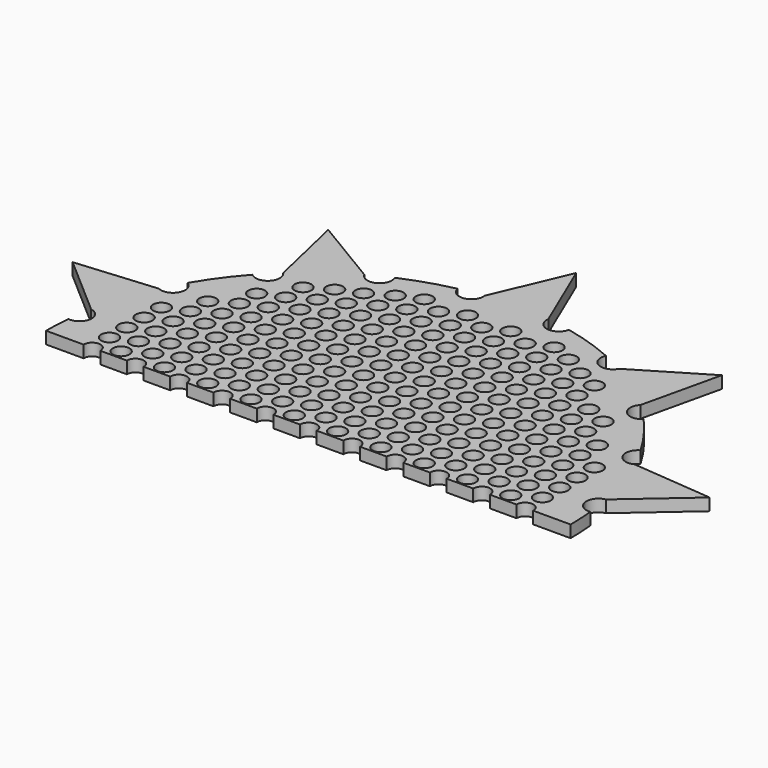
from build123d import *

# Parameters (mm, degrees)
F0_R     = 2.5
F1_DEPTH = 0.127
F3_R     = 0.0875
F4_DEPTH = 0.128
F5_W     = 8.2140588202
F5_H     = 3.6369306035
F6_DEPTH = 25


with BuildPart() as f1:
    # F0 (on Top) → F1 (new body)
    with BuildSketch(Plane.XY):
        with BuildLine():
            ThreePointArc((0.4371819273, 2.5863102989), (0.355691734, 2.6367647524), (0.332670369, 2.7298041002))
            ThreePointArc((0.332670369, 2.7298041002), (0, 2.75), (-0.332670369, 2.7298041002))
            ThreePointArc((-0.332670369, 2.7298041002), (-0.3556917334, 2.6367647532), (-0.4371819253, 2.5863102993))
            ThreePointArc((-0.4371819253, 2.5863102993), (1e-09, 2.623), (0.4371819273, 2.5863102989))
        make_face()
        with BuildLine():
            ThreePointArc((-0.332670369, 2.7298041002), (0, 2.75), (0.332670369, 2.7298041002))
            Line((0.332670369, 2.7298041002), (0, 3.512))
            Line((0, 3.512), (-0.332670369, 2.7298041002))
        make_face()
        with BuildLine():
            ThreePointArc((0.58305072, 2.6874805781), (0.5307280391, 2.6071771648), (0.4371819273, 2.5863102989))
            ThreePointArc((0.4371819273, 2.5863102989), (0.8105515843, 2.4946212396), (1.1665074579, 2.3493380665))
            ThreePointArc((1.1665074579, 2.3493380665), (1.1030922874, 2.4212047401), (1.1079635086, 2.5169260743))
            ThreePointArc((1.1079635086, 2.5169260743), (0.8497967345, 2.6154054198), (0.58305072, 2.6874805781))
        make_face()
        with BuildLine():
            ThreePointArc((1.1665074579, 2.3493380665), (0.8105515843, 2.4946212396), (0.4371819273, 2.5863102989))
            ThreePointArc((0.4371819273, 2.5863102989), (1e-09, 2.623), (-0.4371819253, 2.5863102993))
            ThreePointArc((-0.4371819253, 2.5863102993), (-0.8105515878, 2.4946212385), (-1.1665074663, 2.3493380623))
            ThreePointArc((-1.1665074663, 2.3493380623), (-1.5417607284, 2.1220515678), (-1.8738826621, 1.8353998934))
            ThreePointArc((-1.8738826621, 1.8353998934), (-2.1220515776, 1.5417607149), (-2.3246306188, 1.2149985539))
            ThreePointArc((-2.3246306188, 1.2149985539), (-2.4946212423, 0.8105515762), (-2.5948239078, 0.3834291163))
            ThreePointArc((-2.5948239078, 0.3834291163), (-2.623, 0), (-2.5948239078, -0.3834291163))
            ThreePointArc((-2.5948239078, -0.3834291163), (-2.4946212423, -0.8105515762), (-2.3246306188, -1.2149985539))
            ThreePointArc((-2.3246306188, -1.2149985539), (-2.1220515776, -1.5417607149), (-1.8738826621, -1.8353998934))
            ThreePointArc((-1.8738826621, -1.8353998934), (-1.5417607284, -2.1220515678), (-1.1665074663, -2.3493380623))
            ThreePointArc((-1.1665074663, -2.3493380623), (-0.8105515897, -2.4946212379), (-0.4371819293, -2.5863102986))
            ThreePointArc((-0.4371819293, -2.5863102986), (-1.56e-08, -2.623), (0.4371818986, -2.5863103038))
            ThreePointArc((0.4371818986, -2.5863103038), (0.8105515616, -2.494621247), (1.1665074412, -2.3493380748))
            ThreePointArc((1.1665074412, -2.3493380748), (1.541760707, -2.1220515834), (1.8738826446, -1.8353999112))
            ThreePointArc((1.8738826446, -1.8353999112), (2.1220515703, -1.541760725), (2.3246306188, -1.2149985539))
            ThreePointArc((2.3246306188, -1.2149985539), (2.4946212397, -0.8105515841), (2.5948239054, -0.3834291328))
            ThreePointArc((2.5948239054, -0.3834291328), (2.6159464926, -0.192231496), (2.623, 0))
            ThreePointArc((2.623, 0), (2.6159464926, 0.192231496), (2.5948239054, 0.3834291328))
            ThreePointArc((2.5948239054, 0.3834291328), (2.4946212397, 0.8105515841), (2.3246306188, 1.2149985539))
            ThreePointArc((2.3246306188, 1.2149985539), (2.1220515776, 1.5417607149), (1.8738826621, 1.8353998934))
            ThreePointArc((1.8738826621, 1.8353998934), (1.5417607246, 2.1220515706), (1.1665074579, 2.3493380665))
        make_face()
        Circle(F0_R, mode=Mode.SUBTRACT)
        with BuildLine():
            ThreePointArc((-1.1665074663, 2.3493380623), (-0.8105515878, 2.4946212385), (-0.4371819253, 2.5863102993))
            ThreePointArc((-0.4371819253, 2.5863102993), (-0.5307280383, 2.6071771643), (-0.58305072, 2.6874805781))
            ThreePointArc((-0.58305072, 2.6874805781), (-0.8497967345, 2.6154054198), (-1.1079635086, 2.5169260743))
            ThreePointArc((-1.1079635086, 2.5169260743), (-1.1030922889, 2.4212047357), (-1.1665074663, 2.3493380623))
        make_face()
        with BuildLine():
            ThreePointArc((1.3354026098, 2.4039966451), (1.2620907858, 2.3422578531), (1.1665074579, 2.3493380665))
            ThreePointArc((1.1665074579, 2.3493380665), (1.5417607246, 2.1220515706), (1.8738826621, 1.8353998934))
            ThreePointArc((1.8738826621, 1.8353998934), (1.8376120928, 1.9241171381), (1.8736745738, 2.0129191717))
            ThreePointArc((1.8736745738, 2.0129191717), (1.6164094438, 2.2247967345), (1.3354026098, 2.4039966451))
        make_face()
        with BuildLine():
            ThreePointArc((-1.8738826621, 1.8353998934), (-1.5417607284, 2.1220515678), (-1.1665074663, 2.3493380623))
            ThreePointArc((-1.1665074663, 2.3493380623), (-1.2620907902, 2.3422578545), (-1.3354026098, 2.4039966451))
            ThreePointArc((-1.3354026098, 2.4039966451), (-1.6164094438, 2.2247967345), (-1.8736745738, 2.0129191717))
            ThreePointArc((-1.8736745738, 2.0129191717), (-1.8376120928, 1.9241171381), (-1.8738826621, 1.8353998934))
        make_face()
        with BuildLine():
            ThreePointArc((2.0513593907, 1.8315088452), (1.9618282918, 1.7972965193), (1.8738826621, 1.8353998934))
            ThreePointArc((1.8738826621, 1.8353998934), (2.1220515776, 1.5417607149), (2.3246306188, 1.2149985539))
            ThreePointArc((2.3246306188, 1.2149985539), (2.315568848, 1.3104144102), (2.3757733352, 1.3849913573))
            ThreePointArc((2.3757733352, 1.3849913573), (2.2247967345, 1.6164094438), (2.0513593907, 1.8315088452))
        make_face()
        with BuildLine():
            Line((2.0643018061, 2.8412676842), (1.3354026098, 2.4039966451))
            ThreePointArc((1.3354026098, 2.4039966451), (1.6164094438, 2.2247967345), (1.8736745738, 2.0129191717))
            Line((1.8736745738, 2.0129191717), (2.0643018061, 2.8412676842))
        make_face()
        with BuildLine():
            ThreePointArc((-2.3246306188, 1.2149985539), (-2.1220515776, 1.5417607149), (-1.8738826621, 1.8353998934))
            ThreePointArc((-1.8738826621, 1.8353998934), (-1.9618282918, 1.7972965193), (-2.0513593907, 1.8315088452))
            ThreePointArc((-2.0513593907, 1.8315088452), (-2.2247967345, 1.6164094438), (-2.3757733352, 1.3849913573))
            ThreePointArc((-2.3757733352, 1.3849913573), (-2.315568848, 1.3104144102), (-2.3246306188, 1.2149985539))
        make_face()
        with BuildLine():
            ThreePointArc((-1.8736745738, 2.0129191717), (-1.6164094438, 2.2247967345), (-1.3354026098, 2.4039966451))
            Line((-1.3354026098, 2.4039966451), (-2.0643018061, 2.8412676842))
            Line((-2.0643018061, 2.8412676842), (-1.8736745738, 2.0129191717))
        make_face()
        with BuildLine():
            ThreePointArc((2.4933971802, 1.1599441805), (2.3977975102, 1.1530880597), (2.3246306188, 1.2149985539))
            ThreePointArc((2.3246306188, 1.2149985539), (2.4946212397, 0.8105515841), (2.5948239054, 0.3834291328))
            ThreePointArc((2.5948239054, 0.3834291328), (2.6176270957, 0.4765221848), (2.6989987753, 0.5271675361))
            ThreePointArc((2.6989987753, 0.5271675361), (2.6154054198, 0.8497967345), (2.4933971802, 1.1599441805))
        make_face()
        with BuildLine():
            ThreePointArc((-2.5948239078, 0.3834291163), (-2.4946212423, 0.8105515762), (-2.3246306188, 1.2149985539))
            ThreePointArc((-2.3246306188, 1.2149985539), (-2.3977975102, 1.1530880597), (-2.4933971802, 1.1599441805))
            ThreePointArc((-2.4933971802, 1.1599441805), (-2.6154054198, 0.8497967345), (-2.6989987753, 0.5271675361))
            ThreePointArc((-2.6989987753, 0.5271675361), (-2.6176270909, 0.4765221781), (-2.5948239078, 0.3834291163))
        make_face()
        with BuildLine():
            ThreePointArc((2.7361184973, 0.2759629841), (2.6435768078, 0.300909697), (2.5948239054, 0.3834291328))
            ThreePointArc((2.5948239054, 0.3834291328), (2.6159464926, 0.192231496), (2.623, 0))
            ThreePointArc((2.623, 0), (2.6159464926, -0.192231496), (2.5948239054, -0.3834291328))
            ThreePointArc((2.5948239054, -0.3834291328), (2.6435768078, -0.300909697), (2.7361184973, -0.2759629841))
            ThreePointArc((2.7361184973, -0.2759629841), (2.75, 0), (2.7361184973, 0.2759629841))
        make_face()
        with BuildLine():
            Line((3.3401104852, 1.0852676842), (2.4933971802, 1.1599441805))
            ThreePointArc((2.4933971802, 1.1599441805), (2.6154054198, 0.8497967345), (2.6989987753, 0.5271675361))
            Line((2.6989987753, 0.5271675361), (3.3401104852, 1.0852676842))
        make_face()
        with BuildLine():
            ThreePointArc((-2.5948239078, -0.3834291163), (-2.623, 0), (-2.5948239078, 0.3834291163))
            ThreePointArc((-2.5948239078, 0.3834291163), (-2.6435768144, 0.3009096919), (-2.7361184973, 0.2759629841))
            ThreePointArc((-2.7361184973, 0.2759629841), (-2.75, 0), (-2.7361184973, -0.2759629841))
            ThreePointArc((-2.7361184973, -0.2759629841), (-2.6435768144, -0.3009096919), (-2.5948239078, -0.3834291163))
        make_face()
        with BuildLine():
            ThreePointArc((-2.6989987753, 0.5271675361), (-2.6154054198, 0.8497967345), (-2.4933971802, 1.1599441805))
            Line((-2.4933971802, 1.1599441805), (-3.3401104852, 1.0852676842))
            Line((-3.3401104852, 1.0852676842), (-2.6989987753, 0.5271675361))
        make_face()
        with BuildLine():
            ThreePointArc((-2.3246306188, -1.2149985539), (-2.4946212423, -0.8105515762), (-2.5948239078, -0.3834291163))
            ThreePointArc((-2.5948239078, -0.3834291163), (-2.6176270909, -0.4765221781), (-2.6989987753, -0.5271675361))
            ThreePointArc((-2.6989987753, -0.5271675361), (-2.6154054198, -0.8497967345), (-2.4933971802, -1.1599441805))
            ThreePointArc((-2.4933971802, -1.1599441805), (-2.3977975102, -1.1530880597), (-2.3246306188, -1.2149985539))
        make_face()
        with BuildLine():
            ThreePointArc((2.6989987753, -0.5271675361), (2.6176270957, -0.4765221848), (2.5948239054, -0.3834291328))
            ThreePointArc((2.5948239054, -0.3834291328), (2.4946212397, -0.8105515841), (2.3246306188, -1.2149985539))
            ThreePointArc((2.3246306188, -1.2149985539), (2.3977975102, -1.1530880597), (2.4933971802, -1.1599441805))
            ThreePointArc((2.4933971802, -1.1599441805), (2.6154054198, -0.8497967345), (2.6989987753, -0.5271675361))
        make_face()
        with BuildLine():
            ThreePointArc((-1.8738826621, -1.8353998934), (-2.1220515776, -1.5417607149), (-2.3246306188, -1.2149985539))
            ThreePointArc((-2.3246306188, -1.2149985539), (-2.315568848, -1.3104144102), (-2.3757733352, -1.3849913573))
            ThreePointArc((-2.3757733352, -1.3849913573), (-2.2247967345, -1.6164094438), (-2.0513593907, -1.8315088452))
            ThreePointArc((-2.0513593907, -1.8315088452), (-1.9618282918, -1.7972965193), (-1.8738826621, -1.8353998934))
        make_face()
        with BuildLine():
            ThreePointArc((-2.4933971802, -1.1599441805), (-2.6154054198, -0.8497967345), (-2.6989987753, -0.5271675361))
            Line((-2.6989987753, -0.5271675361), (-3.3401104852, -1.0852676842))
            Line((-3.3401104852, -1.0852676842), (-2.4933971802, -1.1599441805))
        make_face()
        with BuildLine():
            ThreePointArc((2.3757733352, -1.3849913573), (2.315568848, -1.3104144102), (2.3246306188, -1.2149985539))
            ThreePointArc((2.3246306188, -1.2149985539), (2.1220515703, -1.541760725), (1.8738826446, -1.8353999112))
            ThreePointArc((1.8738826446, -1.8353999112), (1.9618282794, -1.7972965196), (2.0513593907, -1.8315088452))
            ThreePointArc((2.0513593907, -1.8315088452), (2.2247967345, -1.6164094438), (2.3757733352, -1.3849913573))
        make_face()
        with BuildLine():
            Line((3.3401104852, -1.0852676842), (2.6989987753, -0.5271675361))
            ThreePointArc((2.6989987753, -0.5271675361), (2.6154054198, -0.8497967345), (2.4933971802, -1.1599441805))
            Line((2.4933971802, -1.1599441805), (3.3401104852, -1.0852676842))
        make_face()
        with BuildLine():
            ThreePointArc((-1.1665074663, -2.3493380623), (-1.5417607284, -2.1220515678), (-1.8738826621, -1.8353998934))
            ThreePointArc((-1.8738826621, -1.8353998934), (-1.8376120928, -1.9241171381), (-1.8736745738, -2.0129191717))
            ThreePointArc((-1.8736745738, -2.0129191717), (-1.6164094438, -2.2247967345), (-1.3354026098, -2.4039966451))
            ThreePointArc((-1.3354026098, -2.4039966451), (-1.2620907902, -2.3422578545), (-1.1665074663, -2.3493380623))
        make_face()
        with BuildLine():
            ThreePointArc((1.8736745738, -2.0129191717), (1.8376120928, -1.9241171506), (1.8738826446, -1.8353999112))
            ThreePointArc((1.8738826446, -1.8353999112), (1.541760707, -2.1220515834), (1.1665074412, -2.3493380748))
            ThreePointArc((1.1665074412, -2.3493380748), (1.2620907769, -2.3422578502), (1.3354026098, -2.4039966451))
            ThreePointArc((1.3354026098, -2.4039966451), (1.6164094438, -2.2247967345), (1.8736745738, -2.0129191717))
        make_face()
        with BuildLine():
            ThreePointArc((-0.4371819293, -2.5863102986), (-0.8105515897, -2.4946212379), (-1.1665074663, -2.3493380623))
            ThreePointArc((-1.1665074663, -2.3493380623), (-1.1030922889, -2.4212047357), (-1.1079635086, -2.5169260743))
            ThreePointArc((-1.1079635086, -2.5169260743), (-0.8497967345, -2.6154054198), (-0.58305072, -2.6874805781))
            ThreePointArc((-0.58305072, -2.6874805781), (-0.5307280399, -2.6071771654), (-0.4371819293, -2.5863102986))
        make_face()
        with BuildLine():
            ThreePointArc((-1.3354026098, -2.4039966451), (-1.6164094438, -2.2247967345), (-1.8736745738, -2.0129191717))
            Line((-1.8736745738, -2.0129191717), (-2.0643018061, -2.8412676842))
            Line((-2.0643018061, -2.8412676842), (-1.3354026098, -2.4039966451))
        make_face()
        with BuildLine():
            ThreePointArc((1.1079635086, -2.5169260743), (1.1030922843, -2.4212047489), (1.1665074412, -2.3493380748))
            ThreePointArc((1.1665074412, -2.3493380748), (0.8105515616, -2.494621247), (0.4371818986, -2.5863103038))
            ThreePointArc((0.4371818986, -2.5863103038), (0.5307280271, -2.6071771565), (0.58305072, -2.6874805781))
            ThreePointArc((0.58305072, -2.6874805781), (0.8497967345, -2.6154054198), (1.1079635086, -2.5169260743))
        make_face()
        with BuildLine():
            Line((2.0643018061, -2.8412676842), (1.8736745738, -2.0129191717))
            ThreePointArc((1.8736745738, -2.0129191717), (1.6164094438, -2.2247967345), (1.3354026098, -2.4039966451))
            Line((1.3354026098, -2.4039966451), (2.0643018061, -2.8412676842))
        make_face()
        with BuildLine():
            ThreePointArc((0.4371818986, -2.5863103038), (-1.56e-08, -2.623), (-0.4371819293, -2.5863102986))
            ThreePointArc((-0.4371819293, -2.5863102986), (-0.3556917345, -2.6367647516), (-0.332670369, -2.7298041002))
            ThreePointArc((-0.332670369, -2.7298041002), (0, -2.75), (0.332670369, -2.7298041002))
            ThreePointArc((0.332670369, -2.7298041002), (0.3556917254, -2.6367647642), (0.4371818986, -2.5863103038))
        make_face()
        with BuildLine():
            ThreePointArc((0.332670369, -2.7298041002), (0, -2.75), (-0.332670369, -2.7298041002))
            Line((-0.332670369, -2.7298041002), (0, -3.512))
            Line((0, -3.512), (0.332670369, -2.7298041002))
        make_face()
        Circle(F0_R)
    extrude(amount=F1_DEPTH)

    # F3 (on offset) → F4 (cut, through all)
    with BuildSketch(Plane.XY.offset(0.127)):
        with Locations((-2.0417519944, 1.2336155081)):
            Circle(F3_R)
        with Locations((-2.0417519944, 1.0066155081)):
            Circle(F3_R)
        with Locations((-2.2690836629, 0.9108655081)):
            Circle(F3_R)
        with Locations((-2.0417519944, 0.7796155081)):
            Circle(F3_R)
        with Locations((-1.5877519944, 1.9146155081)):
            Circle(F3_R)
        with Locations((-1.5877519944, 1.6876155081)):
            Circle(F3_R)
        with Locations((-1.8150836629, 1.5918655081)):
            Circle(F3_R)
        with Locations((-1.5877519944, 1.4606155081)):
            Circle(F3_R)
        with Locations((-1.8150836629, 1.3648655081)):
            Circle(F3_R)
        with Locations((-1.5877519944, 1.2336155081)):
            Circle(F3_R)
        with Locations((-1.8150836629, 1.1378655081)):
            Circle(F3_R)
        with Locations((-1.5877519944, 1.0066155081)):
            Circle(F3_R)
        with Locations((-1.8150836629, 0.9108655081)):
            Circle(F3_R)
        with Locations((-1.5877519944, 0.7796155081)):
            Circle(F3_R)
        with Locations((-1.1337519944, 2.1416155081)):
            Circle(F3_R)
        with Locations((-1.3610836629, 2.0458655081)):
            Circle(F3_R)
        with Locations((-1.1337519944, 1.9146155081)):
            Circle(F3_R)
        with Locations((-1.3610836629, 1.8188655081)):
            Circle(F3_R)
        with Locations((-1.1337519944, 1.6876155081)):
            Circle(F3_R)
        with Locations((-1.3610836629, 1.5918655081)):
            Circle(F3_R)
        with Locations((-1.1337519944, 1.4606155081)):
            Circle(F3_R)
        with Locations((-1.3610836629, 1.3648655081)):
            Circle(F3_R)
        with Locations((-1.1337519944, 1.2336155081)):
            Circle(F3_R)
        with Locations((-1.3610836629, 1.1378655081)):
            Circle(F3_R)
        with Locations((-1.1337519944, 1.0066155081)):
            Circle(F3_R)
        with Locations((-1.3610836629, 0.9108655081)):
            Circle(F3_R)
        with Locations((-1.1337519944, 0.7796155081)):
            Circle(F3_R)
        with Locations((-0.6797519944, 2.3686155081)):
            Circle(F3_R)
        with Locations((-0.9070836629, 2.2728655081)):
            Circle(F3_R)
        with Locations((-0.6797519944, 2.1416155081)):
            Circle(F3_R)
        with Locations((-0.9070836629, 2.0458655081)):
            Circle(F3_R)
        with Locations((-0.6797519944, 1.9146155081)):
            Circle(F3_R)
        with Locations((-0.9070836629, 1.8188655081)):
            Circle(F3_R)
        with Locations((-0.6797519944, 1.6876155081)):
            Circle(F3_R)
        with Locations((-0.9070836629, 1.5918655081)):
            Circle(F3_R)
        with Locations((-0.6797519944, 1.4606155081)):
            Circle(F3_R)
        with Locations((-0.9070836629, 1.3648655081)):
            Circle(F3_R)
        with Locations((-0.6797519944, 1.2336155081)):
            Circle(F3_R)
        with Locations((-0.9070836629, 1.1378655081)):
            Circle(F3_R)
        with Locations((-0.6797519944, 1.0066155081)):
            Circle(F3_R)
        with Locations((-0.9070836629, 0.9108655081)):
            Circle(F3_R)
        with Locations((-0.6797519944, 0.7796155081)):
            Circle(F3_R)
        with Locations((-0.2257519944, 2.3686155081)):
            Circle(F3_R)
        with Locations((-0.4530836629, 2.2728655081)):
            Circle(F3_R)
        with Locations((-0.2257519944, 2.1416155081)):
            Circle(F3_R)
        with Locations((-0.4530836629, 2.0458655081)):
            Circle(F3_R)
        with Locations((-0.2257519944, 1.9146155081)):
            Circle(F3_R)
        with Locations((-0.4530836629, 1.8188655081)):
            Circle(F3_R)
        with Locations((-0.2257519944, 1.6876155081)):
            Circle(F3_R)
        with Locations((-0.4530836629, 1.5918655081)):
            Circle(F3_R)
        with Locations((-0.2257519944, 1.4606155081)):
            Circle(F3_R)
        with Locations((-0.4530836629, 1.3648655081)):
            Circle(F3_R)
        with Locations((-0.2257519944, 1.2336155081)):
            Circle(F3_R)
        with Locations((-0.4530836629, 1.1378655081)):
            Circle(F3_R)
        with Locations((-0.2257519944, 1.0066155081)):
            Circle(F3_R)
        with Locations((-0.4530836629, 0.9108655081)):
            Circle(F3_R)
        with Locations((-0.2257519944, 0.7796155081)):
            Circle(F3_R)
        with Locations((0.2282480056, 2.3686155081)):
            Circle(F3_R)
        with Locations((0.0009163371, 2.2728655081)):
            Circle(F3_R)
        with Locations((0.2282480056, 2.1416155081)):
            Circle(F3_R)
        with Locations((0.0009163371, 2.0458655081)):
            Circle(F3_R)
        with Locations((0.2282480056, 1.9146155081)):
            Circle(F3_R)
        with Locations((0.0009163371, 1.8188655081)):
            Circle(F3_R)
        with Locations((0.2282480056, 1.6876155081)):
            Circle(F3_R)
        with Locations((0.0009163371, 1.5918655081)):
            Circle(F3_R)
        with Locations((0.2282480056, 1.4606155081)):
            Circle(F3_R)
        with Locations((0.0009163371, 1.3648655081)):
            Circle(F3_R)
        with Locations((0.2282480056, 1.2336155081)):
            Circle(F3_R)
        with Locations((0.0009163371, 1.1378655081)):
            Circle(F3_R)
        with Locations((0.2282480056, 1.0066155081)):
            Circle(F3_R)
        with Locations((0.0009163371, 0.9108655081)):
            Circle(F3_R)
        with Locations((0.2282480056, 0.7796155081)):
            Circle(F3_R)
        with Locations((0.6822480056, 2.3686155081)):
            Circle(F3_R)
        with Locations((0.4549163371, 2.2728655081)):
            Circle(F3_R)
        with Locations((0.6822480056, 2.1416155081)):
            Circle(F3_R)
        with Locations((0.4549163371, 2.0458655081)):
            Circle(F3_R)
        with Locations((0.6822480056, 1.9146155081)):
            Circle(F3_R)
        with Locations((0.4549163371, 1.8188655081)):
            Circle(F3_R)
        with Locations((0.6822480056, 1.6876155081)):
            Circle(F3_R)
        with Locations((0.4549163371, 1.5918655081)):
            Circle(F3_R)
        with Locations((0.6822480056, 1.4606155081)):
            Circle(F3_R)
        with Locations((0.4549163371, 1.3648655081)):
            Circle(F3_R)
        with Locations((0.6822480056, 1.2336155081)):
            Circle(F3_R)
        with Locations((0.4549163371, 1.1378655081)):
            Circle(F3_R)
        with Locations((0.6822480056, 1.0066155081)):
            Circle(F3_R)
        with Locations((0.4549163371, 0.9108655081)):
            Circle(F3_R)
        with Locations((0.6822480056, 0.7796155081)):
            Circle(F3_R)
        with Locations((0.9089163371, 2.2728655081)):
            Circle(F3_R)
        with Locations((1.1362480056, 2.1416155081)):
            Circle(F3_R)
        with Locations((0.9089163371, 2.0458655081)):
            Circle(F3_R)
        with Locations((1.1362480056, 1.9146155081)):
            Circle(F3_R)
        with Locations((0.9089163371, 1.8188655081)):
            Circle(F3_R)
        with Locations((1.1362480056, 1.6876155081)):
            Circle(F3_R)
        with Locations((0.9089163371, 1.5918655081)):
            Circle(F3_R)
        with Locations((1.1362480056, 1.4606155081)):
            Circle(F3_R)
        with Locations((0.9089163371, 1.3648655081)):
            Circle(F3_R)
        with Locations((1.1362480056, 1.2336155081)):
            Circle(F3_R)
        with Locations((0.9089163371, 1.1378655081)):
            Circle(F3_R)
        with Locations((1.1362480056, 1.0066155081)):
            Circle(F3_R)
        with Locations((0.9089163371, 0.9108655081)):
            Circle(F3_R)
        with Locations((1.1362480056, 0.7796155081)):
            Circle(F3_R)
        with Locations((1.3629163371, 2.0458655081)):
            Circle(F3_R)
        with Locations((1.3629163371, 1.8188655081)):
            Circle(F3_R)
        with Locations((1.5902480056, 1.6876155081)):
            Circle(F3_R)
        with Locations((1.3629163371, 1.5918655081)):
            Circle(F3_R)
        with Locations((1.5902480056, 1.4606155081)):
            Circle(F3_R)
        with Locations((1.3629163371, 1.3648655081)):
            Circle(F3_R)
        with Locations((1.5902480056, 1.2336155081)):
            Circle(F3_R)
        with Locations((1.3629163371, 1.1378655081)):
            Circle(F3_R)
        with Locations((1.5902480056, 1.0066155081)):
            Circle(F3_R)
        with Locations((1.3629163371, 0.9108655081)):
            Circle(F3_R)
        with Locations((1.5902480056, 0.7796155081)):
            Circle(F3_R)
        with Locations((1.8169163371, 1.5918655081)):
            Circle(F3_R)
        with Locations((1.8169163371, 1.3648655081)):
            Circle(F3_R)
        with Locations((2.0442480056, 1.2336155081)):
            Circle(F3_R)
        with Locations((1.8169163371, 1.1378655081)):
            Circle(F3_R)
        with Locations((2.0442480056, 1.0066155081)):
            Circle(F3_R)
        with Locations((1.8169163371, 0.9108655081)):
            Circle(F3_R)
        with Locations((2.0442480056, 0.7796155081)):
            Circle(F3_R)
        with Locations((-2.2690836629, 0.6838655081)):
            Circle(F3_R)
        with Locations((-2.0417519944, 0.5526155081)):
            Circle(F3_R)
        with Locations((-2.2690836629, 0.4568655081)):
            Circle(F3_R)
        with Locations((-2.0417519944, 0.3256155081)):
            Circle(F3_R)
        with Locations((-2.2690836629, 0.2298655081)):
            Circle(F3_R)
        with Locations((-2.0417519944, 0.0986155081)):
            Circle(F3_R)
        with Locations((-2.2690836629, 0.0028655081)):
            Circle(F3_R)
        with Locations((-2.0417519944, -0.1283844919)):
            Circle(F3_R)
        with Locations((-2.2690836629, -0.2241344919)):
            Circle(F3_R)
        with Locations((-2.0417519944, -0.3553844919)):
            Circle(F3_R)
        with Locations((-2.2690836629, -0.4511344919)):
            Circle(F3_R)
        with Locations((-2.0417519944, -0.5823844919)):
            Circle(F3_R)
        with Locations((-2.2690836629, -0.6781344919)):
            Circle(F3_R)
        with Locations((-2.0417519944, -0.8093844919)):
            Circle(F3_R)
        with Locations((-2.2690836629, -0.9051344919)):
            Circle(F3_R)
        with Locations((-2.0417519944, -1.0363844919)):
            Circle(F3_R)
        with Locations((-2.0417519944, -1.2633844919)):
            Circle(F3_R)
        with Locations((-1.8150836629, 0.6838655081)):
            Circle(F3_R)
        with Locations((-1.5877519944, 0.5526155081)):
            Circle(F3_R)
        with Locations((-1.8150836629, 0.4568655081)):
            Circle(F3_R)
        with Locations((-1.5877519944, 0.3256155081)):
            Circle(F3_R)
        with Locations((-1.8150836629, 0.2298655081)):
            Circle(F3_R)
        with Locations((-1.5877519944, 0.0986155081)):
            Circle(F3_R)
        with Locations((-1.8150836629, 0.0028655081)):
            Circle(F3_R)
        with Locations((-1.5877519944, -0.1283844919)):
            Circle(F3_R)
        with Locations((-1.8150836629, -0.2241344919)):
            Circle(F3_R)
        with Locations((-1.5877519944, -0.3553844919)):
            Circle(F3_R)
        with Locations((-1.8150836629, -0.4511344919)):
            Circle(F3_R)
        with Locations((-1.5877519944, -0.5823844919)):
            Circle(F3_R)
        with Locations((-1.8150836629, -0.6781344919)):
            Circle(F3_R)
        with Locations((-1.5877519944, -0.8093844919)):
            Circle(F3_R)
        with Locations((-1.8150836629, -0.9051344919)):
            Circle(F3_R)
        with Locations((-1.5877519944, -1.0363844919)):
            Circle(F3_R)
        with Locations((-1.8150836629, -1.1321344919)):
            Circle(F3_R)
        with Locations((-1.5877519944, -1.2633844919)):
            Circle(F3_R)
        with Locations((-1.8150836629, -1.3591344919)):
            Circle(F3_R)
        with Locations((-1.5877519944, -1.4903844919)):
            Circle(F3_R)
        with Locations((-1.8150836629, -1.5861344919)):
            Circle(F3_R)
        with Locations((-1.5877519944, -1.7173844919)):
            Circle(F3_R)
        with Locations((-1.3610836629, 0.6838655081)):
            Circle(F3_R)
        with Locations((-1.1337519944, 0.5526155081)):
            Circle(F3_R)
        with Locations((-1.3610836629, 0.4568655081)):
            Circle(F3_R)
        with Locations((-1.1337519944, 0.3256155081)):
            Circle(F3_R)
        with Locations((-1.3610836629, 0.2298655081)):
            Circle(F3_R)
        with Locations((-1.1337519944, 0.0986155081)):
            Circle(F3_R)
        with Locations((-1.3610836629, 0.0028655081)):
            Circle(F3_R)
        with Locations((-1.1337519944, -0.1283844919)):
            Circle(F3_R)
        with Locations((-1.3610836629, -0.2241344919)):
            Circle(F3_R)
        with Locations((-1.1337519944, -0.3553844919)):
            Circle(F3_R)
        with Locations((-1.3610836629, -0.4511344919)):
            Circle(F3_R)
        with Locations((-1.1337519944, -0.5823844919)):
            Circle(F3_R)
        with Locations((-1.3610836629, -0.6781344919)):
            Circle(F3_R)
        with Locations((-1.1337519944, -0.8093844919)):
            Circle(F3_R)
        with Locations((-1.3610836629, -0.9051344919)):
            Circle(F3_R)
        with Locations((-1.1337519944, -1.0363844919)):
            Circle(F3_R)
        with Locations((-1.3610836629, -1.1321344919)):
            Circle(F3_R)
        with Locations((-1.1337519944, -1.2633844919)):
            Circle(F3_R)
        with Locations((-1.3610836629, -1.3591344919)):
            Circle(F3_R)
        with Locations((-1.1337519944, -1.4903844919)):
            Circle(F3_R)
        with Locations((-1.3610836629, -1.5861344919)):
            Circle(F3_R)
        with Locations((-1.1337519944, -1.7173844919)):
            Circle(F3_R)
        with Locations((-0.9070836629, 0.6838655081)):
            Circle(F3_R)
        with Locations((-0.6797519944, 0.5526155081)):
            Circle(F3_R)
        with Locations((-0.9070836629, 0.4568655081)):
            Circle(F3_R)
        with Locations((-0.6797519944, 0.3256155081)):
            Circle(F3_R)
        with Locations((-0.9070836629, 0.2298655081)):
            Circle(F3_R)
        with Locations((-0.6797519944, 0.0986155081)):
            Circle(F3_R)
        with Locations((-0.9070836629, 0.0028655081)):
            Circle(F3_R)
        with Locations((-0.6797519944, -0.1283844919)):
            Circle(F3_R)
        with Locations((-0.9070836629, -0.2241344919)):
            Circle(F3_R)
        with Locations((-0.6797519944, -0.3553844919)):
            Circle(F3_R)
        with Locations((-0.9070836629, -0.4511344919)):
            Circle(F3_R)
        with Locations((-0.6797519944, -0.5823844919)):
            Circle(F3_R)
        with Locations((-0.9070836629, -0.6781344919)):
            Circle(F3_R)
        with Locations((-0.6797519944, -0.8093844919)):
            Circle(F3_R)
        with Locations((-0.9070836629, -0.9051344919)):
            Circle(F3_R)
        with Locations((-0.6797519944, -1.0363844919)):
            Circle(F3_R)
        with Locations((-0.9070836629, -1.1321344919)):
            Circle(F3_R)
        with Locations((-0.6797519944, -1.2633844919)):
            Circle(F3_R)
        with Locations((-0.9070836629, -1.3591344919)):
            Circle(F3_R)
        with Locations((-0.6797519944, -1.4903844919)):
            Circle(F3_R)
        with Locations((-0.9070836629, -1.5861344919)):
            Circle(F3_R)
        with Locations((-0.6797519944, -1.7173844919)):
            Circle(F3_R)
        with Locations((-0.4530836629, 0.6838655081)):
            Circle(F3_R)
        with Locations((-0.2257519944, 0.5526155081)):
            Circle(F3_R)
        with Locations((-0.4530836629, 0.4568655081)):
            Circle(F3_R)
        with Locations((-0.2257519944, 0.3256155081)):
            Circle(F3_R)
        with Locations((-0.4530836629, 0.2298655081)):
            Circle(F3_R)
        with Locations((-0.2257519944, 0.0986155081)):
            Circle(F3_R)
        with Locations((-0.4530836629, 0.0028655081)):
            Circle(F3_R)
        with Locations((-0.2257519944, -0.1283844919)):
            Circle(F3_R)
        with Locations((-0.4530836629, -0.2241344919)):
            Circle(F3_R)
        with Locations((-0.2257519944, -0.3553844919)):
            Circle(F3_R)
        with Locations((-0.4530836629, -0.4511344919)):
            Circle(F3_R)
        with Locations((-0.2257519944, -0.5823844919)):
            Circle(F3_R)
        with Locations((-0.4530836629, -0.6781344919)):
            Circle(F3_R)
        with Locations((-0.2257519944, -0.8093844919)):
            Circle(F3_R)
        with Locations((-0.4530836629, -0.9051344919)):
            Circle(F3_R)
        with Locations((-0.2257519944, -1.0363844919)):
            Circle(F3_R)
        with Locations((-0.4530836629, -1.1321344919)):
            Circle(F3_R)
        with Locations((-0.2257519944, -1.2633844919)):
            Circle(F3_R)
        with Locations((-0.4530836629, -1.3591344919)):
            Circle(F3_R)
        with Locations((-0.2257519944, -1.4903844919)):
            Circle(F3_R)
        with Locations((-0.4530836629, -1.5861344919)):
            Circle(F3_R)
        with Locations((-0.2257519944, -1.7173844919)):
            Circle(F3_R)
        with Locations((0.0009163371, 0.6838655081)):
            Circle(F3_R)
        with Locations((0.2282480056, 0.5526155081)):
            Circle(F3_R)
        with Locations((0.0009163371, 0.4568655081)):
            Circle(F3_R)
        with Locations((0.2282480056, 0.3256155081)):
            Circle(F3_R)
        with Locations((0.0009163371, 0.2298655081)):
            Circle(F3_R)
        with Locations((0.2282480056, 0.0986155081)):
            Circle(F3_R)
        with Locations((0.0009163371, 0.0028655081)):
            Circle(F3_R)
        with Locations((0.2282480056, -0.1283844919)):
            Circle(F3_R)
        with Locations((0.0009163371, -0.2241344919)):
            Circle(F3_R)
        with Locations((0.2282480056, -0.3553844919)):
            Circle(F3_R)
        with Locations((0.0009163371, -0.4511344919)):
            Circle(F3_R)
        with Locations((0.2282480056, -0.5823844919)):
            Circle(F3_R)
        with Locations((0.0009163371, -0.6781344919)):
            Circle(F3_R)
        with Locations((0.2282480056, -0.8093844919)):
            Circle(F3_R)
        with Locations((0.0009163371, -0.9051344919)):
            Circle(F3_R)
        with Locations((0.2282480056, -1.0363844919)):
            Circle(F3_R)
        with Locations((0.0009163371, -1.1321344919)):
            Circle(F3_R)
        with Locations((0.2282480056, -1.2633844919)):
            Circle(F3_R)
        with Locations((0.0009163371, -1.3591344919)):
            Circle(F3_R)
        with Locations((0.2282480056, -1.4903844919)):
            Circle(F3_R)
        with Locations((0.0009163371, -1.5861344919)):
            Circle(F3_R)
        with Locations((0.2282480056, -1.7173844919)):
            Circle(F3_R)
        with Locations((0.4549163371, 0.6838655081)):
            Circle(F3_R)
        with Locations((0.6822480056, 0.5526155081)):
            Circle(F3_R)
        with Locations((0.4549163371, 0.4568655081)):
            Circle(F3_R)
        with Locations((0.6822480056, 0.3256155081)):
            Circle(F3_R)
        with Locations((0.4549163371, 0.2298655081)):
            Circle(F3_R)
        with Locations((0.6822480056, 0.0986155081)):
            Circle(F3_R)
        with Locations((0.4549163371, 0.0028655081)):
            Circle(F3_R)
        with Locations((0.6822480056, -0.1283844919)):
            Circle(F3_R)
        with Locations((0.4549163371, -0.2241344919)):
            Circle(F3_R)
        with Locations((0.6822480056, -0.3553844919)):
            Circle(F3_R)
        with Locations((0.4549163371, -0.4511344919)):
            Circle(F3_R)
        with Locations((0.6822480056, -0.5823844919)):
            Circle(F3_R)
        with Locations((0.4549163371, -0.6781344919)):
            Circle(F3_R)
        with Locations((0.6822480056, -0.8093844919)):
            Circle(F3_R)
        with Locations((0.4549163371, -0.9051344919)):
            Circle(F3_R)
        with Locations((0.6822480056, -1.0363844919)):
            Circle(F3_R)
        with Locations((0.4549163371, -1.1321344919)):
            Circle(F3_R)
        with Locations((0.6822480056, -1.2633844919)):
            Circle(F3_R)
        with Locations((0.4549163371, -1.3591344919)):
            Circle(F3_R)
        with Locations((0.6822480056, -1.4903844919)):
            Circle(F3_R)
        with Locations((0.4549163371, -1.5861344919)):
            Circle(F3_R)
        with Locations((0.6822480056, -1.7173844919)):
            Circle(F3_R)
        with Locations((0.9089163371, 0.6838655081)):
            Circle(F3_R)
        with Locations((1.1362480056, 0.5526155081)):
            Circle(F3_R)
        with Locations((0.9089163371, 0.4568655081)):
            Circle(F3_R)
        with Locations((1.1362480056, 0.3256155081)):
            Circle(F3_R)
        with Locations((0.9089163371, 0.2298655081)):
            Circle(F3_R)
        with Locations((1.1362480056, 0.0986155081)):
            Circle(F3_R)
        with Locations((0.9089163371, 0.0028655081)):
            Circle(F3_R)
        with Locations((1.1362480056, -0.1283844919)):
            Circle(F3_R)
        with Locations((0.9089163371, -0.2241344919)):
            Circle(F3_R)
        with Locations((1.1362480056, -0.3553844919)):
            Circle(F3_R)
        with Locations((0.9089163371, -0.4511344919)):
            Circle(F3_R)
        with Locations((1.1362480056, -0.5823844919)):
            Circle(F3_R)
        with Locations((0.9089163371, -0.6781344919)):
            Circle(F3_R)
        with Locations((1.1362480056, -0.8093844919)):
            Circle(F3_R)
        with Locations((0.9089163371, -0.9051344919)):
            Circle(F3_R)
        with Locations((1.1362480056, -1.0363844919)):
            Circle(F3_R)
        with Locations((0.9089163371, -1.1321344919)):
            Circle(F3_R)
        with Locations((1.1362480056, -1.2633844919)):
            Circle(F3_R)
        with Locations((0.9089163371, -1.3591344919)):
            Circle(F3_R)
        with Locations((1.1362480056, -1.4903844919)):
            Circle(F3_R)
        with Locations((0.9089163371, -1.5861344919)):
            Circle(F3_R)
        with Locations((1.1362480056, -1.7173844919)):
            Circle(F3_R)
        with Locations((1.3629163371, 0.6838655081)):
            Circle(F3_R)
        with Locations((1.5902480056, 0.5526155081)):
            Circle(F3_R)
        with Locations((1.3629163371, 0.4568655081)):
            Circle(F3_R)
        with Locations((1.5902480056, 0.3256155081)):
            Circle(F3_R)
        with Locations((1.3629163371, 0.2298655081)):
            Circle(F3_R)
        with Locations((1.5902480056, 0.0986155081)):
            Circle(F3_R)
        with Locations((1.3629163371, 0.0028655081)):
            Circle(F3_R)
        with Locations((1.5902480056, -0.1283844919)):
            Circle(F3_R)
        with Locations((1.3629163371, -0.2241344919)):
            Circle(F3_R)
        with Locations((1.5902480056, -0.3553844919)):
            Circle(F3_R)
        with Locations((1.3629163371, -0.4511344919)):
            Circle(F3_R)
        with Locations((1.5902480056, -0.5823844919)):
            Circle(F3_R)
        with Locations((1.3629163371, -0.6781344919)):
            Circle(F3_R)
        with Locations((1.5902480056, -0.8093844919)):
            Circle(F3_R)
        with Locations((1.3629163371, -0.9051344919)):
            Circle(F3_R)
        with Locations((1.5902480056, -1.0363844919)):
            Circle(F3_R)
        with Locations((1.3629163371, -1.1321344919)):
            Circle(F3_R)
        with Locations((1.5902480056, -1.2633844919)):
            Circle(F3_R)
        with Locations((1.3629163371, -1.3591344919)):
            Circle(F3_R)
        with Locations((1.5902480056, -1.4903844919)):
            Circle(F3_R)
        with Locations((1.3629163371, -1.5861344919)):
            Circle(F3_R)
        with Locations((1.5902480056, -1.7173844919)):
            Circle(F3_R)
        with Locations((1.8169163371, 0.6838655081)):
            Circle(F3_R)
        with Locations((2.0442480056, 0.5526155081)):
            Circle(F3_R)
        with Locations((1.8169163371, 0.4568655081)):
            Circle(F3_R)
        with Locations((2.0442480056, 0.3256155081)):
            Circle(F3_R)
        with Locations((1.8169163371, 0.2298655081)):
            Circle(F3_R)
        with Locations((2.0442480056, 0.0986155081)):
            Circle(F3_R)
        with Locations((1.8169163371, 0.0028655081)):
            Circle(F3_R)
        with Locations((2.0442480056, -0.1283844919)):
            Circle(F3_R)
        with Locations((1.8169163371, -0.2241344919)):
            Circle(F3_R)
        with Locations((2.0442480056, -0.3553844919)):
            Circle(F3_R)
        with Locations((1.8169163371, -0.4511344919)):
            Circle(F3_R)
        with Locations((2.0442480056, -0.5823844919)):
            Circle(F3_R)
        with Locations((1.8169163371, -0.6781344919)):
            Circle(F3_R)
        with Locations((2.0442480056, -0.8093844919)):
            Circle(F3_R)
        with Locations((1.8169163371, -0.9051344919)):
            Circle(F3_R)
        with Locations((2.0442480056, -1.0363844919)):
            Circle(F3_R)
        with Locations((1.8169163371, -1.1321344919)):
            Circle(F3_R)
        with Locations((2.0442480056, -1.2633844919)):
            Circle(F3_R)
        with Locations((1.8169163371, -1.3591344919)):
            Circle(F3_R)
        with Locations((1.8169163371, -1.5861344919)):
            Circle(F3_R)
        with Locations((2.2709163371, 0.9108655081)):
            Circle(F3_R)
        with Locations((2.2709163371, 0.6838655081)):
            Circle(F3_R)
        with Locations((2.2709163371, 0.4568655081)):
            Circle(F3_R)
        with Locations((2.2709163371, 0.2298655081)):
            Circle(F3_R)
        with Locations((2.2709163371, 0.0028655081)):
            Circle(F3_R)
        with Locations((2.2709163371, -0.2241344919)):
            Circle(F3_R)
        with Locations((2.2709163371, -0.4511344919)):
            Circle(F3_R)
        with Locations((2.2709163371, -0.6781344919)):
            Circle(F3_R)
        with Locations((2.2709163371, -0.9051344919)):
            Circle(F3_R)
        with Locations((-1.3610836629, -1.8131344919)):
            Circle(F3_R)
        with Locations((-1.1337519944, -1.9443844919)):
            Circle(F3_R)
        with Locations((-1.3610836629, -2.0401344919)):
            Circle(F3_R)
        with Locations((-1.1337519944, -2.1713844919)):
            Circle(F3_R)
        with Locations((-0.9070836629, -1.8131344919)):
            Circle(F3_R)
        with Locations((-0.6797519944, -1.9443844919)):
            Circle(F3_R)
        with Locations((-0.9070836629, -2.0401344919)):
            Circle(F3_R)
        with Locations((-0.6797519944, -2.1713844919)):
            Circle(F3_R)
        with Locations((-0.9070836629, -2.2671344919)):
            Circle(F3_R)
        with Locations((-0.4530836629, -1.8131344919)):
            Circle(F3_R)
        with Locations((-0.2257519944, -1.9443844919)):
            Circle(F3_R)
        with Locations((-0.4530836629, -2.0401344919)):
            Circle(F3_R)
        with Locations((-0.2257519944, -2.1713844919)):
            Circle(F3_R)
        with Locations((-0.4530836629, -2.2671344919)):
            Circle(F3_R)
        with Locations((-0.2257519944, -2.3983844919)):
            Circle(F3_R)
        with Locations((0.0009163371, -1.8131344919)):
            Circle(F3_R)
        with Locations((0.2282480056, -1.9443844919)):
            Circle(F3_R)
        with Locations((0.0009163371, -2.0401344919)):
            Circle(F3_R)
        with Locations((0.2282480056, -2.1713844919)):
            Circle(F3_R)
        with Locations((0.0009163371, -2.2671344919)):
            Circle(F3_R)
        with Locations((0.2282480056, -2.3983844919)):
            Circle(F3_R)
        with Locations((0.4549163371, -1.8131344919)):
            Circle(F3_R)
        with Locations((0.6822480056, -1.9443844919)):
            Circle(F3_R)
        with Locations((0.4549163371, -2.0401344919)):
            Circle(F3_R)
        with Locations((0.6822480056, -2.1713844919)):
            Circle(F3_R)
        with Locations((0.4549163371, -2.2671344919)):
            Circle(F3_R)
        with Locations((0.9089163371, -1.8131344919)):
            Circle(F3_R)
        with Locations((1.1362480056, -1.9443844919)):
            Circle(F3_R)
        with Locations((0.9089163371, -2.0401344919)):
            Circle(F3_R)
        with Locations((1.1362480056, -2.1713844919)):
            Circle(F3_R)
        with Locations((0.9089163371, -2.2671344919)):
            Circle(F3_R)
        with Locations((1.3629163371, -1.8131344919)):
            Circle(F3_R)
        with Locations((1.3629163371, -2.0401344919)):
            Circle(F3_R)
    extrude(amount=-F4_DEPTH, mode=Mode.SUBTRACT)

    # F5 (on face) → F6 (cut)
    with BuildSketch(Plane.XY.offset(0.127)):
        with Locations((0.0718256924, -1.8184653018)):
            Rectangle(F5_W, F5_H)
    extrude(amount=-F6_DEPTH, mode=Mode.SUBTRACT)


solid = f1.part
